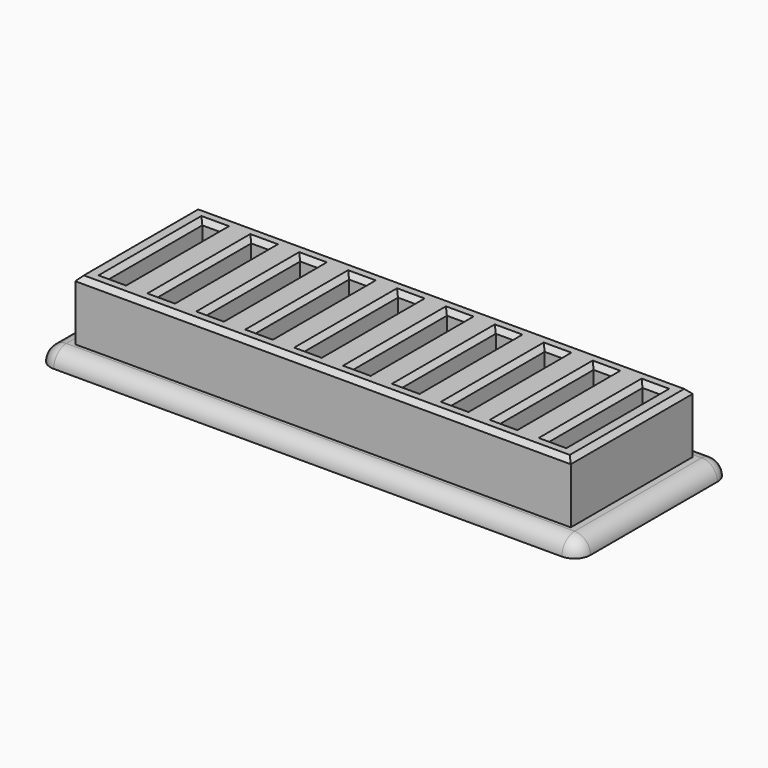
from build123d import *

# Parameters (mm, degrees)
F0_W     = 156
F0_H     = 48
F1_DEPTH = 2
F2_W     = 156
F2_H     = 48
F2_W_2   = 5.7
F2_H_2   = 37.5
F3_DEPTH = 22
F0_W_2   = 170
F0_H_2   = 60
F4_DEPTH = 5
F5_R     = 4.99999
F6_SIZE  = 1.5


# Not quite as in the source:
# - a fillet or chamfer is up to 0.001 mm smaller than in the source, because OpenCascade refuses the exact size


with BuildPart() as f1:
    # F0 (on Top) → F1 (new body)
    with BuildSketch(Plane.XY):
        Rectangle(F0_W, F0_H)
    extrude(amount=F1_DEPTH)

    # F2 (on face) → F3 (join)
    with BuildSketch(Plane.XY.offset(2)):
        Rectangle(F2_W, F2_H)
        with Locations((-69.35, 0)):
            Rectangle(F2_W_2, F2_H_2, mode=Mode.SUBTRACT)
        with Locations((-53.95, 0)):
            Rectangle(F2_W_2, F2_H_2, mode=Mode.SUBTRACT)
        with Locations((-38.55, 0)):
            Rectangle(F2_W_2, F2_H_2, mode=Mode.SUBTRACT)
        with Locations((-23.15, 0)):
            Rectangle(F2_W_2, F2_H_2, mode=Mode.SUBTRACT)
        with Locations((-7.75, 0)):
            Rectangle(F2_W_2, F2_H_2, mode=Mode.SUBTRACT)
        with Locations((7.65, 0)):
            Rectangle(F2_W_2, F2_H_2, mode=Mode.SUBTRACT)
        with Locations((23.05, 0)):
            Rectangle(F2_W_2, F2_H_2, mode=Mode.SUBTRACT)
        with Locations((38.45, 0)):
            Rectangle(F2_W_2, F2_H_2, mode=Mode.SUBTRACT)
        with Locations((53.85, 0)):
            Rectangle(F2_W_2, F2_H_2, mode=Mode.SUBTRACT)
        with Locations((69.25, 0)):
            Rectangle(F2_W_2, F2_H_2, mode=Mode.SUBTRACT)
    extrude(amount=F3_DEPTH)

    # F0 (on Top) → F4 (join)
    with BuildSketch(Plane.XY):
        Rectangle(F0_W_2, F0_H_2)
        Rectangle(F0_W, F0_H, mode=Mode.SUBTRACT)
    extrude(amount=F4_DEPTH)

    # F5 (radius 5 in the source; OpenCascade refuses exactly that, so slightly less here)
    f5_edges = [f1.edges().sort_by_distance(p)[0] for p in [
        (0, -30, 5),
        (-85, 0, 5),
        (0, 30, 5),
        (85, 0, 5),
        (85, -30, 2.5),
        (85, 30, 2.5),
        (-85, -30, 2.5),
        (-85, 30, 2.5),
    ]]
    fillet(f5_edges, radius=F5_R)

    # F6
    f6_edges = [f1.edges().sort_by_distance(p)[0] for p in [
        (0, -24, 24),
        (-78, 0, 24),
        (0, 24, 24),
        (78, 0, 24),
        (-72.2, 0, 24),
        (-66.5, 0, 24),
        (-69.35, -18.75, 24),
        (-69.35, 18.75, 24),
        (-53.95, -18.75, 24),
        (-51.1, 0, 24),
        (-56.8, 0, 24),
        (-53.95, 18.75, 24),
        (-38.55, 18.75, 24),
        (-41.4, 0, 24),
        (-38.55, -18.75, 24),
        (-35.7, 0, 24),
        (-26, 0, 24),
        (-20.3, 0, 24),
        (-23.15, -18.75, 24),
        (-23.15, 18.75, 24),
        (-10.6, 0, 24),
        (-7.75, 18.75, 24),
        (-4.9, 0, 24),
        (-7.75, -18.75, 24),
        (7.65, -18.75, 24),
        (4.8, 0, 24),
        (10.5, 0, 24),
        (7.65, 18.75, 24),
        (20.2, 0, 24),
        (23.05, 18.75, 24),
        (25.9, 0, 24),
        (23.05, -18.75, 24),
        (38.45, -18.75, 24),
        (35.6, 0, 24),
        (41.3, 0, 24),
        (38.45, 18.75, 24),
        (51, 0, 24),
        (53.85, -18.75, 24),
        (56.7, 0, 24),
        (53.85, 18.75, 24),
        (66.4, 0, 24),
        (69.25, -18.75, 24),
        (72.1, 0, 24),
        (69.25, 18.75, 24),
    ]]
    chamfer(f6_edges, length=F6_SIZE)


solid = f1.part
